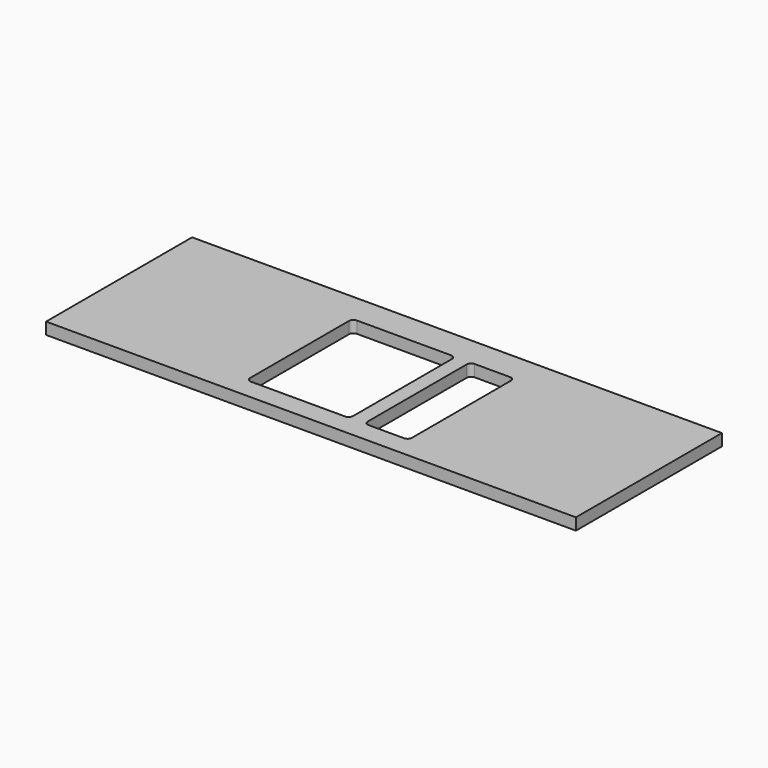
from build123d import *

# Parameters (mm, degrees)
F0_W     = 620
F0_H     = 40
F1_DEPTH = 1800
F3_DEPTH = 40.001


# Not quite as in the source:
# - a feature of the source that left no trace in its solid (it failed there, or was rolled back) is left out


with BuildPart() as f1:
    # F0 (on Right) → F1 (new body)
    with BuildSketch(Plane.YZ):
        with Locations((-310, 20)):
            Rectangle(F0_W, F0_H)
    extrude(amount=F1_DEPTH)

    # F2 (on face) → F3 (cut, through all)
    with BuildSketch(Plane.XY.offset(40)):
        with BuildLine():
            Line((960, -100), (640, -100))
            ThreePointArc((640, -100), (629.3933982822, -104.3933982822), (625, -115))
            Line((625, -115), (625, -535))
            ThreePointArc((625, -535), (629.3933982822, -545.6066017178), (640, -550))
            Line((640, -550), (960, -550))
            ThreePointArc((960, -550), (970.6066017178, -545.6066017178), (975, -535))
            Line((975, -535), (975, -115))
            ThreePointArc((975, -115), (970.6066017178, -104.3933982822), (960, -100))
        make_face()
        with BuildLine():
            Line((1160, -100), (1040, -100))
            ThreePointArc((1040, -100), (1029.3933982822, -104.3933982822), (1025, -115))
            Line((1025, -115), (1025, -535))
            ThreePointArc((1025, -535), (1029.3933982822, -545.6066017178), (1040, -550))
            Line((1040, -550), (1160, -550))
            ThreePointArc((1160, -550), (1170.6066017178, -545.6066017178), (1175, -535))
            Line((1175, -535), (1175, -115))
            ThreePointArc((1175, -115), (1170.6066017178, -104.3933982822), (1160, -100))
        make_face()
    extrude(amount=-F3_DEPTH, mode=Mode.SUBTRACT)


solid = f1.part
